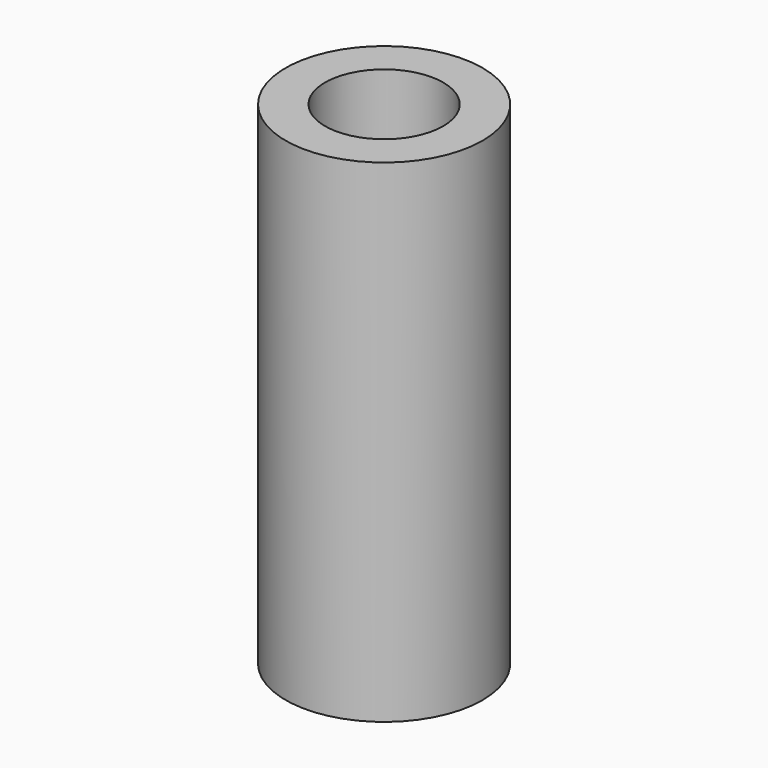
from build123d import *

# Parameters (mm, degrees)
F0_R       = 50
F1_DEPTH   = 200
F2_R       = 30
F3_DEPTH   = 150
F1_FACE1_R = 50
F4_R       = 10
F5_DEPTH   = 50
F6_R       = 10
F7_DEPTH   = 150
F8_W       = 25
F8_H       = 25
F8_R       = 10
F9_DEPTH   = 50


# Not quite as in the source:
# - a fillet or chamfer that OpenCascade refuses, or shapes differently, is made with other operations: its cross-section is extruded or revolved along the edge and cut away or added


with BuildPart() as f1:
    # F0 (on Top) → F1 (new body)
    with BuildSketch(Plane.XY):
        Circle(F0_R)
    extrude(amount=F1_DEPTH)

    # F2 (on face) → F3 (cut)
    with BuildSketch(Plane.XY.offset(200)):
        Circle(F2_R)
    extrude(amount=-F3_DEPTH, mode=Mode.SUBTRACT)

    # F1_face1 (on face) + F4 (on face) → F5 (join)
    with BuildSketch(Plane(origin=(0, 0, 0), x_dir=(1, 0, 0), z_dir=(0, 0, -1))):
        Circle(F1_FACE1_R)
    with BuildSketch(Plane(origin=(0, 0, 0), x_dir=(1, 0, 0), z_dir=(0, 0, -1))):
        Circle(F4_R)
    extrude(amount=F5_DEPTH)

    # F6 (on face) → F7 (cut)
    with BuildSketch(Plane(origin=(0, 0, -50), x_dir=(1, 0, 0), z_dir=(0, 0, -1))):
        Circle(F6_R)
    extrude(amount=-F7_DEPTH, mode=Mode.SUBTRACT)

    # F8 (on face) → F9 (join)
    with BuildSketch(Plane.XY.offset(50)):
        Rectangle(F8_W, F8_H)
        Circle(F8_R, mode=Mode.SUBTRACT)
    extrude(amount=F9_DEPTH)

    # F10: chamfer of 15 on 1 edges, made by hand

    # F10_s1 → F10_t2 (revolve)
    with BuildSketch(Plane.XZ):
        Polygon((30, 65), (15, 50), (30, 50), align=None)
    revolve(axis=Axis((0, 0, 50), (0, 0, 1)))


solid = f1.part
